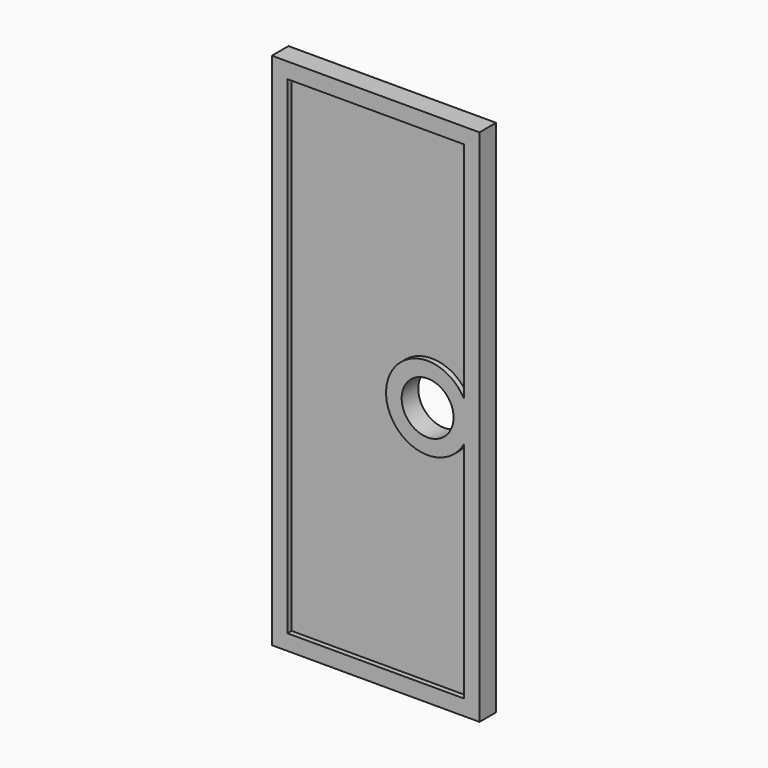
from build123d import *

# Parameters (mm, degrees)
F0_W         = 20
F0_H         = 50
F0_R         = 2.5
F1_DEPTH     = 1
F2_T         = -1.5
F3_T         = 1
F3_T3_DEPTH  = 23.5635083269
F3_T5_DEPTH  = 2.5
F3_T7_DEPTH  = 23.5635083269
F3_T9_DEPTH  = 19
F3_T11_DEPTH = 49
F3_T14_ANGLE = 302.0899512573


# Not quite as in the source:
# - a shell that OpenCascade refuses in one call is made with other operations: the cavity is built on its own and cut out


with BuildPart() as f1:
    # F0 (on Front) → F1 (new body, symmetric)
    with BuildSketch(Plane.XZ):
        Rectangle(F0_W, F0_H)
        with Locations((5, 0)):
            Circle(F0_R, mode=Mode.SUBTRACT)
    extrude(amount=F1_DEPTH, both=True)

    # F2
    f2_openings = [f1.faces().sort_by_distance(p)[0] for p in [
        (-0.100141, -1, 0),
    ]]
    offset(amount=F2_T, openings=f2_openings, kind=Kind.INTERSECTION)

    # F3: shell of thickness 1, made by hand


with BuildPart() as f3_core1:
    # F3_t2: copy of F1
    add(f1.part)

    # the walls: a layer under each face that stays
    f3_faces = [f3_core1.faces().sort_by_distance(p)[0] for p in [
        (10, 0, 0),
        (0, 0, -25),
        (-10, 0, 0),
        (0, 0, 25),
        (2.5, 0, 0),
        (-8.5714285714, -1, -21.4285714286),
        (8.5, -0.75, 12.7182458366),
        (8.5, -0.75, -12.7182458366),
        (0, -0.75, -23.5),
        (-8.5, -0.75, 0),
        (1, -0.75, 0),
        (0, -0.75, 23.5),
        (0, -0.5, 0),
    ]]
    thicken(f3_faces, amount=-F3_T, mode=Mode.SUBTRACT)

    # F3_s4 → F3_t3 (cut)
    with BuildSketch(Plane.XY.offset(0.9364916731)):
        Polygon((8.49, -0.51), (9.5, -0.5), (9.5, 0.5), (8.5, 0.5), align=None)
    extrude(amount=F3_T3_DEPTH, mode=Mode.SUBTRACT)

    # F3_s6 → F3_t5 (cut)
    with BuildSketch(Plane.XZ.offset(-0.5)):
        Polygon((8.49, 23.49), (9.5, 23.5), (9.5, 24.5), (8.5, 24.5), align=None)
        Polygon((8.49875, 1.9413329023), (9.5, 1.9364916731), (9.5, -1.9364916731), (7.625, 1.4523687548), align=None)
        Polygon((8.49, -23.49), (9.5, -23.5), (9.5, -24.5), (8.5, -24.5), align=None)
        Polygon((8.49875, -1.9413329023), (9.5, -1.9364916731), (9.5, 1.9364916731), (7.625, -1.4523687548), align=None)
        Polygon((-8.49, -23.49), (-8.5, -24.5), (-9.5, -24.5), (-9.5, -23.5), align=None)
        Polygon((-8.49, 23.49), (-9.5, 23.5), (-9.5, 24.5), (-8.5, 24.5), align=None)
    extrude(amount=F3_T5_DEPTH, mode=Mode.SUBTRACT)

    # F3_s8 → F3_t7 (cut)
    with BuildSketch(Plane.XY.offset(-24.5)):
        Polygon((8.49, -0.51), (9.5, -0.5), (9.5, 0.5), (8.5, 0.5), align=None)
    extrude(amount=F3_T7_DEPTH, mode=Mode.SUBTRACT)

    # F3_s10 → F3_t9 (cut)
    with BuildSketch(Plane.YZ.offset(-9.5)):
        Polygon((-0.51, -23.49), (-0.5, -24.5), (0.5, -24.5), (0.5, -23.5), align=None)
        Polygon((-0.51, 23.49), (-0.5, 24.5), (0.5, 24.5), (0.5, 23.5), align=None)
    extrude(amount=F3_T9_DEPTH, mode=Mode.SUBTRACT)

    # F3_s12 → F3_t11 (cut)
    with BuildSketch(Plane.XY.offset(-24.5)):
        Polygon((-8.49, -0.51), (-9.5, -0.5), (-9.5, 0.5), (-8.5, 0.5), align=None)
    extrude(amount=F3_T11_DEPTH, mode=Mode.SUBTRACT)

    # F3_s13 → F3_t14 (revolve, cut)
    with BuildSketch(Plane(origin=(1.171875, 0, 2.1180377675), x_dir=(0, 1, 0), z_dir=(0.4841229183, 0, 0.875))):
        Polygon((-0.51, -8.385), (-0.5, -7.375), (0.5, -7.375), (0.5, -8.375), align=None)
    revolve(axis=Axis((5, -0.5, 0), (0, 1, 0)), revolution_arc=F3_T14_ANGLE, mode=Mode.SUBTRACT)


with BuildPart() as f1_1:
    add(f1.part)

    # what is left inside the walls is the cavity
    f3_cavity = [f3_core1.part.solids().sort_by_distance(p)[0] for p in [
        (0, 0.99, -8),
    ]]
    add(f3_cavity, mode=Mode.SUBTRACT)


solid = f1_1.part
